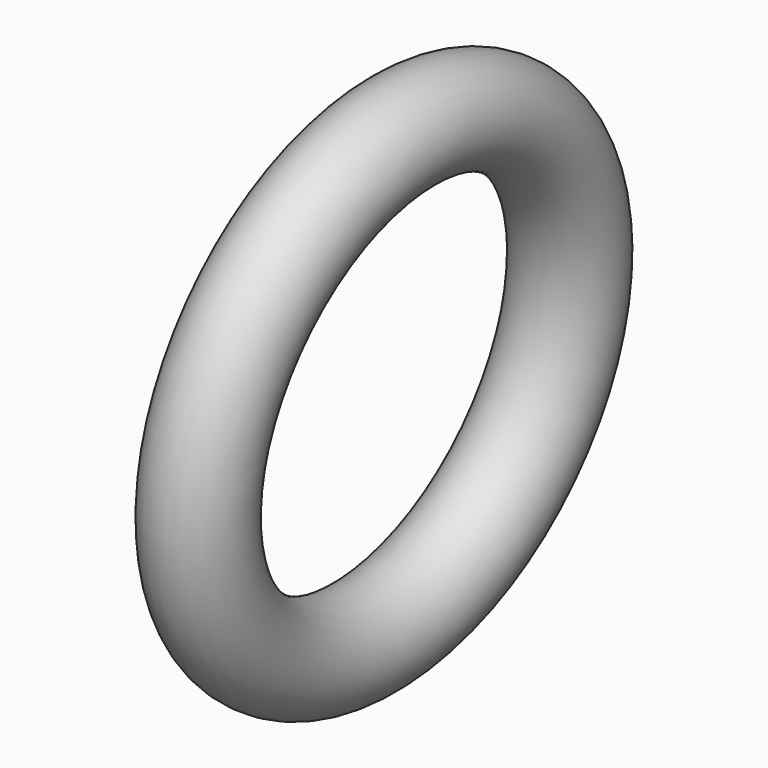
from build123d import *

# Parameters (mm, degrees)
F2_R = 15.3678554399


# Not quite as in the source:
# - the program builds the solid bodies; features that only make, move or delete a surface that nothing else refers to are left out


with BuildPart() as f3:
    # F2 (on Front) → F3 (revolve)
    with BuildSketch(Plane.XZ):
        with Locations((-65.6882598996, 39.254900068)):
            Circle(F2_R)
    revolve(axis=Axis((-7.423649542, 0, -38.5525841266), (0.9962153136, 0, -0.0869197845)))


solid = f3.part
